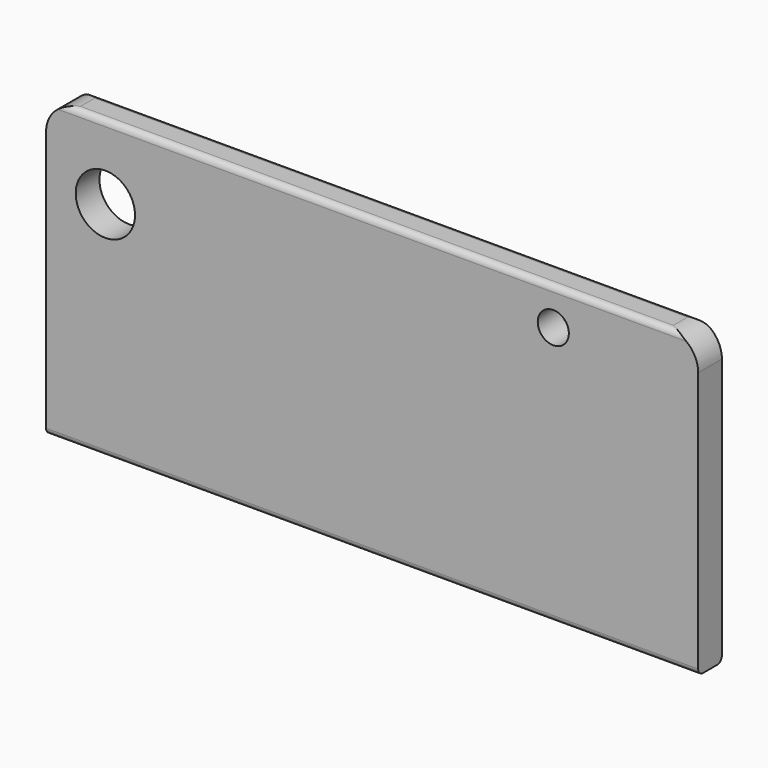
from build123d import *

# Parameters (mm, degrees)
F0_R        = 10
F1_DEPTH    = 10
F2_T1_DEPTH = 217
F2_T3_DEPTH = 230
F4_D        = 10.5


# Not quite as in the source:
# - a fillet or chamfer that OpenCascade refuses, or shapes differently, is made with other operations: its cross-section is extruded or revolved along the edge and cut away or added


with BuildPart() as f1:
    # F0 (on Front) → F1 (new body)
    with BuildSketch(Plane.XZ):
        with BuildLine():
            Line((0, 90), (0, 0))
            Line((0, 0), (220, 0))
            Line((220, 0), (220, 90))
            ThreePointArc((220, 90), (217.0710678119, 97.0710678119), (210, 100))
            Line((210, 100), (10, 100))
            ThreePointArc((10, 100), (2.9289321881, 97.0710678119), (0, 90))
        make_face()
        with Locations((20, 75)):
            Circle(F0_R, mode=Mode.SUBTRACT)
    extrude(amount=F1_DEPTH)

    # F2: fillet of radius 2 on 4 edges, made by hand

    # F2_s2 → F2_t1 (cut)
    with BuildSketch(Plane.YZ.offset(1.5)):
        with BuildLine():
            ThreePointArc((-8, 100), (-9.4142135624, 99.4142135624), (-10, 98))
            Line((-10, 98), (-10, 100))
            Line((-10, 100), (-8, 100))
        make_face()
        with BuildLine():
            ThreePointArc((-2, 100), (-0.5857864376, 99.4142135624), (0, 98))
            Line((0, 98), (0, 100))
            Line((0, 100), (-2, 100))
        make_face()
    extrude(amount=F2_T1_DEPTH, mode=Mode.SUBTRACT)

    # F2_s4 → F2_t3 (cut)
    with BuildSketch(Plane.YZ.offset(-5)):
        with BuildLine():
            ThreePointArc((-8, 0), (-9.4142135624, 0.5857864376), (-10, 2))
            Line((-10, 2), (-10, 0))
            Line((-10, 0), (-8, 0))
        make_face()
        with BuildLine():
            ThreePointArc((-2, 0), (-0.5857864376, 0.5857864376), (0, 2))
            Line((0, 2), (0, 0))
            Line((0, 0), (-2, 0))
        make_face()
    extrude(amount=F2_T3_DEPTH, mode=Mode.SUBTRACT)

    # F4 (through all)
    with Locations(Plane.XZ.offset(10)):
        with Locations((171.1133077741, 87.5)):
            Hole(F4_D / 2)


solid = f1.part
